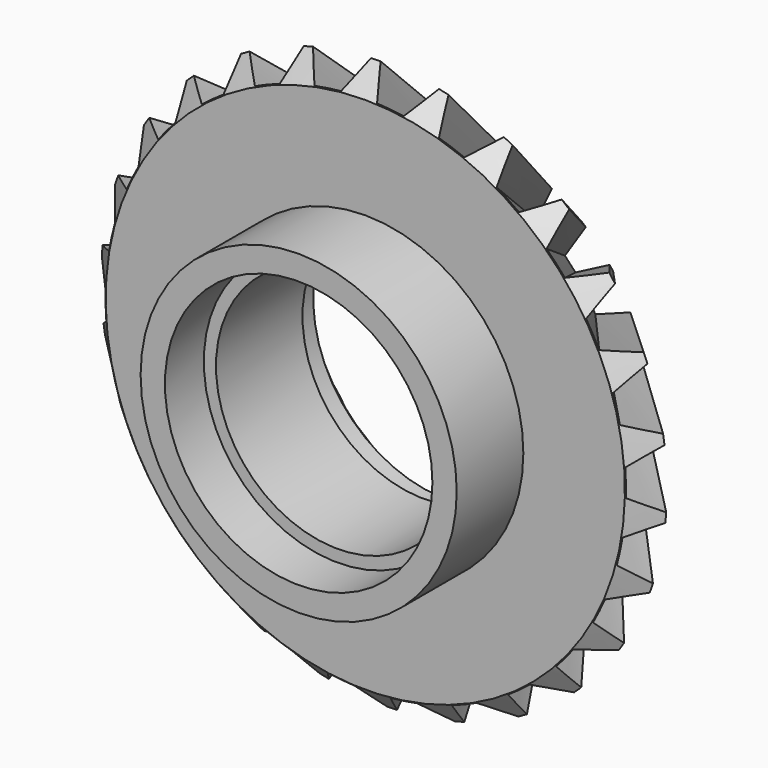
from build123d import *

# Parameters (mm, degrees)
F4_R      = 65
F5_DEPTH  = 34.25
F6_R      = 55
F6_R_2    = 50
F7_DEPTH  = 20
F9_R      = 55
F9_R_2    = 50
F10_DEPTH = 73
F11_DEPTH = 333


# Not quite as in the source:
# - ends of sketch curves that miss each other by under 0.0002 mm in the source are joined


with BuildPart() as f3:
    # F0 (on Front) → F3 section 0
    with BuildSketch(Plane.XZ):
        with BuildLine():
            Line((4.647425, 107.14926), (-1.469582, 125.991429))
            ThreePointArc((-1.469582, 125.991429), (-3.6339068263, 125.9475871987), (-5.7971590014, 125.8665680295))
            Line((-5.7971590014, 125.8665680295), (-10.196493, 106.764198))
            ThreePointArc((-10.196493, 106.764198), (-15.6841394295, 106.0969852086), (-21.1301169921, 105.1478989609))
            Line((-21.1301169921, 105.1478989609), (-31.578602, 121.978653))
            ThreePointArc((-31.578602, 121.978653), (-33.6695433104, 121.4181281904), (-35.7505460521, 120.8217631761))
            Line((-35.7505460521, 120.8217631761), (-35.450546, 101.221644))
            ThreePointArc((-35.450546, 101.221644), (-40.6190569723, 99.2605395446), (-45.6796531382, 97.0357242936))
            Line((-45.6796531382, 97.0357242936), (-59.852387, 110.876921))
            ThreePointArc((-59.852387, 110.876921), (-61.7484272238, 109.8322891293), (-63.626240453, 108.7552367742))
            Line((-63.626240453, 108.7552367742), (-58.644343, 89.796456))
            ThreePointArc((-58.644343, 89.796456), (-63.1933432848, 86.6554318233), (-67.5744545742, 83.2841857077))
            Line((-67.5744545742, 83.2841857077), (-84.64777, 93.331425))
            ThreePointArc((-84.64777, 93.331425), (-86.2387176403, 91.8633963), (-87.8042092574, 90.3682512649))
            Line((-87.8042092574, 90.3682512649), (-78.429944, 73.152624))
            ThreePointArc((-78.429944, 73.152624), (-82.0950620329, 69.0142252714), (-85.5420740481, 64.6924730363))
            Line((-85.5420740481, 64.6924730363), (-104.523732, 70.361846))
            ThreePointArc((-104.523732, 70.361846), (-105.7171271923, 68.5557365814), (-106.8793169138, 66.7293909462))
            Line((-106.8793169138, 66.7293909462), (-93.657481, 52.257427))
            ThreePointArc((-93.657481, 52.257427), (-96.2257139986, 47.3621628039), (-98.5382990262, 42.3410690113))
            Line((-98.5382990262, 42.3410690113), (-118.325154, 43.303093))
            ThreePointArc((-118.325154, 43.303093), (-119.0516411498, 41.2638672394), (-119.7429867773, 39.2124612546))
            Line((-119.7429867773, 39.2124612546), (-103.441986, 28.325219))
            ThreePointArc((-103.441986, 28.325219), (-104.764077079, 22.9575837968), (-105.8078361957, 17.5289560324))
            Line((-105.8078361957, 17.5289560324), (-125.249949, 13.727721))
            ThreePointArc((-125.249949, 13.727721), (-125.4673066239, 11.5738916766), (-125.6476294147, 9.4166460311))
            Line((-125.6476294147, 9.4166460311), (-107.214818, 2.746852))
            ThreePointArc((-107.214818, 2.746852), (-107.2139328185, -2.7812064998), (-106.9282065415, -8.301876042))
            Line((-106.9282065415, -8.301876042), (-124.895671, -16.645457))
            ThreePointArc((-124.895671, -16.645457), (-124.5912682706, -18.7887165799), (-124.2500886239, -20.9264301051))
            Line((-124.2500886239, -20.9264301051), (-104.756715, -22.991152))
            ThreePointArc((-104.756715, -22.991152), (-103.4329044086, -28.3583635916), (-101.8342980115, -33.6502340038))
            Line((-101.8342980115, -33.6502340038), (-117.282912, -46.051261))
            ThreePointArc((-117.282912, -46.051261), (-116.4744381713, -48.0593929703), (-115.6315841333, -50.0533390577))
            Line((-115.6315841333, -50.0533390577), (-96.210533, -47.392994))
            ThreePointArc((-96.210533, -47.392994), (-93.6407315432, -52.2874353555), (-90.8221502197, -57.042962138))
            Line((-90.8221502197, -57.042962138), (-102.854096, -72.780733))
            ThreePointArc((-102.854096, -72.780733), (-101.588537404, -74.537031522), (-100.2929927716, -76.2713288263))
            Line((-100.2929927716, -76.2713288263), (-82.072944, -69.040527))
            ThreePointArc((-82.072944, -69.040527), (-78.4065001697, -73.1777509298), (-74.5317498938, -77.1205598901))
            Line((-74.5317498938, -77.1205598901), (-82.447773, -95.280453))
            ThreePointArc((-82.447773, -95.280453), (-80.7986798888, -96.6828491938), (-79.1257368917, -98.0567068657))
            Line((-79.1257368917, -98.0567068657), (-63.165574, -86.675676))
            ThreePointArc((-63.165574, -86.675676), (-58.6155674419, -89.8152423226), (-53.9098340917, -92.7161921576))
            Line((-53.9098340917, -92.7161921576), (-57.249886, -112.24282))
            ThreePointArc((-57.249886, -112.24282), (-55.3130968687, -113.2098110359), (-53.359980765, -114.1433854972))
            Line((-53.359980765, -114.1433854972), (-40.58725, -99.27355))
            ThreePointArc((-40.58725, -99.27355), (-35.4181109459, -101.2329981628), (-30.1548749802, -102.9234959323))
            Line((-30.1548749802, -102.9234959323), (-28.724843, -122.682042))
            ThreePointArc((-28.724843, -122.682042), (-26.6129171945, -123.1574303012), (-24.4931359084, -123.5964655376))
            Line((-24.4931359084, -123.5964655376), (-15.650143, -106.102006))
            ThreePointArc((-15.650143, -106.102006), (-10.1622832517, -106.7674599263), (-4.6474249612, -107.1492601058))
            Line((-4.6474249612, -107.1492601058), (1.469583, -125.99143))
            ThreePointArc((1.469583, -125.99143), (3.6339078195, -125.9475871701), (5.7971599992, -125.8665679835))
            Line((5.7971599992, -125.8665679835), (10.196493, -106.764199))
            ThreePointArc((10.196493, -106.764199), (15.6841393825, -106.0969852156), (21.1301169921, -105.1478989609))
            Line((21.1301169921, -105.1478989609), (31.578602, -121.978654))
            ThreePointArc((31.578602, -121.978654), (33.6695430529, -121.4181282618), (35.75054578, -120.8217632566))
            Line((35.75054578, -120.8217632566), (35.450547, -101.221645))
            ThreePointArc((35.450547, -101.221645), (40.6190574777, -99.2605393378), (45.6796535714, -97.0357240896))
            Line((45.6796535714, -97.0357240896), (59.852388, -110.876922))
            ThreePointArc((59.852388, -110.876922), (61.7484275564, -109.8322889423), (63.6262407621, -108.7552365934))
            Line((63.6262407621, -108.7552365934), (58.644343, -89.796456))
            ThreePointArc((58.644343, -89.796456), (63.193343344, -86.6554317802), (67.574454688, -83.2841856154))
            Line((67.574454688, -83.2841856154), (84.64777, -93.331426))
            ThreePointArc((84.64777, -93.331426), (86.2387174028, -91.8633965229), (87.804209272, -90.3682512507))
            Line((87.804209272, -90.3682512507), (78.429944, -73.152625))
            ThreePointArc((78.429944, -73.152625), (82.095061541, -69.0142258565), (85.5420735669, -64.6924736725))
            Line((85.5420735669, -64.6924736725), (104.523732, -70.361847))
            ThreePointArc((104.523732, -70.361847), (105.7171267358, -68.5557372853), (106.8793164645, -66.7293916657))
            Line((106.8793164645, -66.7293916657), (93.657481, -52.257428))
            ThreePointArc((93.657481, -52.257428), (96.2257136029, -47.3621636079), (98.5382986635, -42.3410698554))
            Line((98.5382986635, -42.3410698554), (118.325154, -43.303093))
            ThreePointArc((118.325154, -43.303093), (119.0516410451, -41.2638675413), (119.7429865784, -39.212461862))
            Line((119.7429865784, -39.212461862), (103.441986, -28.32522))
            ThreePointArc((103.441986, -28.32522), (104.7640768702, -22.9575847497), (105.8078360344, -17.5289570057))
            Line((105.8078360344, -17.5289570057), (125.249949, -13.727721))
            ThreePointArc((125.249949, -13.727721), (125.4673065815, -11.5738921359), (125.6476293457, -9.416646951))
            Line((125.6476293457, -9.416646951), (107.214819, -2.746853))
            ThreePointArc((107.214819, -2.746853), (107.2139328321, 2.7812059742), (106.9282065475, 8.3018759649))
            Line((106.9282065475, 8.3018759649), (124.895672, 16.645456))
            ThreePointArc((124.895672, 16.645456), (124.5912683668, 18.7887159424), (124.2500886515, 20.9264299413))
            Line((124.2500886515, 20.9264299413), (104.756716, 22.991151))
            ThreePointArc((104.756716, 22.991151), (103.4329046917, 28.3583625593), (101.8342983094, 33.6502331022))
            Line((101.8342983094, 33.6502331022), (117.282912, 46.05126))
            ThreePointArc((117.282912, 46.05126), (116.4744385996, 48.0593919323), (115.6315846557, 50.0533378509))
            Line((115.6315846557, 50.0533378509), (96.210533, 47.392993))
            ThreePointArc((96.210533, 47.392993), (93.6407320979, 52.287434362), (90.822150953, 57.0429609705))
            Line((90.822150953, 57.0429609705), (102.854096, 72.780732))
            ThreePointArc((102.854096, 72.780732), (101.5885378809, 74.537030872), (100.2929932534, 76.2713281927))
            Line((100.2929932534, 76.2713281927), (82.072944, 69.040526))
            ThreePointArc((82.072944, 69.040526), (78.4065004308, 73.17775065), (74.5317498938, 77.1205598901))
            Line((74.5317498938, 77.1205598901), (82.447774, 95.280452))
            ThreePointArc((82.447774, 95.280452), (80.7986806709, 96.6828485402), (79.1257373804, 98.0567064714))
            Line((79.1257373804, 98.0567064714), (63.165574, 86.675675))
            ThreePointArc((63.165574, 86.675675), (58.6155682609, 89.8152417881), (53.9098352735, 92.7161914704))
            Line((53.9098352735, 92.7161914704), (57.249886, 112.242819))
            ThreePointArc((57.249886, 112.242819), (55.3130972631, 113.2098108432), (53.3599811486, 114.1433853179))
            Line((53.3599811486, 114.1433853179), (40.587251, 99.273549))
            ThreePointArc((40.587251, 99.273549), (35.418112147, 101.2329977425), (30.1548761709, 102.9234955834))
            Line((30.1548761709, 102.9234955834), (28.724844, 122.682041))
            ThreePointArc((28.724844, 122.682041), (26.6129183562, 123.1574300502), (24.4931370613, 123.5964653091))
            Line((24.4931370613, 123.5964653091), (15.650144, 106.102005))
            ThreePointArc((15.650144, 106.102005), (10.1622838383, 106.7674598705), (4.647425, 107.14926))
        make_face()
    # F2 (on offset) → F3 section 1
    with BuildSketch(Plane.XZ.offset(-56.5685)):
        with BuildLine():
            Line((-19.7001110751, 66.5780655763), (-18.0915129272, 51.6565431383))
            ThreePointArc((-18.0915129272, 51.6565431383), (-20.7291642653, 50.655730553), (-23.3117433893, 49.5203383384))
            Line((-23.3117433893, 49.5203383384), (-32.9812778687, 61.0980237192))
            ThreePointArc((-32.9812778687, 61.0980237192), (-34.0260786064, 60.5223856678), (-35.0608356411, 59.9288828229))
            Line((-35.0608356411, 59.9288828229), (-29.9280263775, 45.8259154425))
            ThreePointArc((-29.9280263775, 45.8259154425), (-32.2495222328, 44.2229533699), (-34.485339159, 42.502501951))
            Line((-34.485339159, 42.502501951), (-46.6446160079, 51.4296897689))
            ThreePointArc((-46.6446160079, 51.4296897689), (-47.5212975323, 50.6207415305), (-48.3839518806, 49.7968512324))
            Line((-48.3839518806, 49.7968512324), (-40.0252317187, 37.3320521117))
            ThreePointArc((-40.0252317187, 37.3320521117), (-41.8956551903, 35.2200988808), (-43.6547723658, 33.0145746404))
            Line((-43.6547723658, 33.0145746404), (-57.597138611, 38.7724491885))
            ThreePointArc((-57.597138611, 38.7724491885), (-58.2547513786, 37.7772038943), (-58.8951687053, 36.7708076526))
            Line((-58.8951687053, 36.7708076526), (-47.7963160781, 26.6685856085))
            ThreePointArc((-47.7963160781, 26.6685856085), (-49.1069649527, 24.1703802647), (-50.2871488814, 21.6079602549))
            Line((-50.2871488814, 21.6079602549), (-65.2023248751, 23.8618947934))
            ThreePointArc((-65.2023248751, 23.8618947934), (-65.6026508221, 22.7381924823), (-65.9836124001, 21.6077783884))
            Line((-65.9836124001, 21.6077783884), (-52.7896522797, 14.4552378462))
            ThreePointArc((-52.7896522797, 14.4552378462), (-53.4643564085, 11.7159670033), (-53.9970190904, 8.945569761))
            Line((-53.9970190904, 8.945569761), (-69.0181890183, 7.5645738073))
            ThreePointArc((-69.0181890183, 7.5645738073), (-69.1379626558, 6.3777199733), (-69.2373283829, 5.1889835853))
            Line((-69.2373283829, 5.1889835853), (-54.7150457733, 1.4018042029))
            ThreePointArc((-54.7150457733, 1.4018042029), (-54.714593805, -1.4193356746), (-54.568778821, -4.2367047315))
            Line((-54.568778821, -4.2367047315), (-68.8229668866, -9.1723727123))
            ThreePointArc((-68.8229668866, -9.1723727123), (-68.6552274062, -10.3534024386), (-68.4672225075, -11.5313760825))
            Line((-68.4672225075, -11.5313760825), (-53.4605996877, -11.7330972054))
            ThreePointArc((-53.4605996877, -11.7330972054), (-52.7850178889, -14.4721517221), (-51.969199476, -17.1727573448))
            Line((-51.969199476, -17.1727573448), (-64.6280040808, -25.3762542701))
            ThreePointArc((-64.6280040808, -25.3762542701), (-64.1824998913, -26.4828227338), (-63.7180505282, -27.5815740873))
            Line((-63.7180505282, -27.5815740873), (-49.0992178696, -24.1861136521))
            ThreePointArc((-49.0992178696, -24.1861136521), (-47.7877685989, -26.6838989156), (-46.3493591578, -29.1107917217))
            Line((-46.3493591578, -29.1107917217), (-56.6770965911, -40.1053601686))
            ThreePointArc((-56.6770965911, -40.1053601686), (-55.9797187767, -41.0731576329), (-55.2658170579, -42.0288312611))
            Line((-55.2658170579, -42.0288312611), (-41.8843679773, -35.2335210863))
            ThreePointArc((-41.8843679773, -35.2335210863), (-40.0132678994, -37.3448748962), (-38.0358625584, -39.3570126971))
            Line((-38.0358625584, -39.3570126971), (-45.4323222603, -52.5036883112))
            ThreePointArc((-45.4323222603, -52.5036883112), (-44.5235998847, -53.2764699051), (-43.6017351833, -54.0335255305))
            Line((-43.6017351833, -54.0335255305), (-32.2353508617, -44.2332843436))
            ThreePointArc((-32.2353508617, -44.2332843436), (-29.9133415119, -45.8355024909), (-27.5118598818, -47.3159471515))
            Line((-27.5118598818, -47.3159471515), (-31.5471864996, -61.8506929323))
            ThreePointArc((-31.5471864996, -61.8506929323), (-30.4799312042, -62.3835473986), (-29.4036789456, -62.8979877))
            Line((-29.4036789456, -62.8979877), (-20.7129323247, -50.6623698963))
            ThreePointArc((-20.7129323247, -50.6623698963), (-18.0749604462, -51.6623372861), (-15.3889679105, -52.5250507439))
            Line((-15.3889679105, -52.5250507439), (-15.8286429288, -67.6031600983))
            ThreePointArc((-15.8286429288, -67.6031600983), (-14.6648797121, -67.8651198723), (-13.4967877657, -68.1070474493))
            Line((-13.4967877657, -68.1070474493), (-7.9867534495, -54.1471426609))
            ThreePointArc((-7.9867534495, -54.1471426609), (-5.1861283793, -54.4867448232), (-2.3717250608, -54.6815893079))
            Line((-2.3717250608, -54.6815893079), (0.8098038342, -69.4267773269))
            ThreePointArc((0.8098038342, -69.4267773269), (2.0024412842, -69.4026182586), (3.1944876603, -69.3579731598))
            Line((3.1944876603, -69.3579731598), (5.2035865056, -54.4850803108))
            ThreePointArc((5.2035865056, -54.4850803108), (8.0041026182, -54.1445808025), (10.7833538285, -53.6602326608))
            Line((10.7833538285, -53.6602326608), (17.4011877418, -67.2155626133))
            ThreePointArc((17.4011877418, -67.2155626133), (18.5533876716, -66.90668874), (19.7001110751, -66.5780655763))
            Line((19.7001110751, -66.5780655763), (18.0915129272, -51.6565431383))
            ThreePointArc((18.0915129272, -51.6565431383), (20.7291642653, -50.655730553), (23.3117433893, -49.5203383384))
            Line((23.3117433893, -49.5203383384), (32.9812778687, -61.0980237192))
            ThreePointArc((32.9812778687, -61.0980237192), (34.0260786064, -60.5223856678), (35.0608356411, -59.9288828229))
            Line((35.0608356411, -59.9288828229), (29.9280263775, -45.8259154425))
            ThreePointArc((29.9280263775, -45.8259154425), (32.2495222328, -44.2229533699), (34.485339159, -42.502501951))
            Line((34.485339159, -42.502501951), (46.6446160079, -51.4296897689))
            ThreePointArc((46.6446160079, -51.4296897689), (47.5212975323, -50.6207415305), (48.3839518806, -49.7968512324))
            Line((48.3839518806, -49.7968512324), (40.0252317187, -37.3320521117))
            ThreePointArc((40.0252317187, -37.3320521117), (41.8956551903, -35.2200988808), (43.6547723658, -33.0145746404))
            Line((43.6547723658, -33.0145746404), (57.597138611, -38.7724491885))
            ThreePointArc((57.597138611, -38.7724491885), (58.2547513786, -37.7772038943), (58.8951687053, -36.7708076526))
            Line((58.8951687053, -36.7708076526), (47.7963160781, -26.6685856085))
            ThreePointArc((47.7963160781, -26.6685856085), (49.1069649527, -24.1703802647), (50.2871488814, -21.6079602549))
            Line((50.2871488814, -21.6079602549), (65.2023248751, -23.8618947934))
            ThreePointArc((65.2023248751, -23.8618947934), (65.6026508221, -22.7381924823), (65.9836124001, -21.6077783884))
            Line((65.9836124001, -21.6077783884), (52.7896522797, -14.4552378462))
            ThreePointArc((52.7896522797, -14.4552378462), (53.4643564085, -11.7159670033), (53.9970190904, -8.945569761))
            Line((53.9970190904, -8.945569761), (69.0181890183, -7.5645738073))
            ThreePointArc((69.0181890183, -7.5645738073), (69.1379626558, -6.3777199733), (69.2373283829, -5.1889835853))
            Line((69.2373283829, -5.1889835853), (54.7150457733, -1.4018042029))
            ThreePointArc((54.7150457733, -1.4018042029), (54.714593805, 1.4193356746), (54.568778821, 4.2367047315))
            Line((54.568778821, 4.2367047315), (68.8229668866, 9.1723727123))
            ThreePointArc((68.8229668866, 9.1723727123), (68.6552274062, 10.3534024386), (68.4672225075, 11.5313760825))
            Line((68.4672225075, 11.5313760825), (53.4605996877, 11.7330972054))
            ThreePointArc((53.4605996877, 11.7330972054), (52.7850178889, 14.4721517221), (51.969199476, 17.1727573448))
            Line((51.969199476, 17.1727573448), (64.6280040808, 25.3762542701))
            ThreePointArc((64.6280040808, 25.3762542701), (64.1824998913, 26.4828227338), (63.7180505282, 27.5815740873))
            Line((63.7180505282, 27.5815740873), (49.0992178696, 24.1861136521))
            ThreePointArc((49.0992178696, 24.1861136521), (47.7877685989, 26.6838989156), (46.3493591578, 29.1107917217))
            Line((46.3493591578, 29.1107917217), (56.6770965911, 40.1053601686))
            ThreePointArc((56.6770965911, 40.1053601686), (55.9797187767, 41.0731576329), (55.2658170579, 42.0288312611))
            Line((55.2658170579, 42.0288312611), (41.8843679773, 35.2335210863))
            ThreePointArc((41.8843679773, 35.2335210863), (40.0132678994, 37.3448748962), (38.0358625584, 39.3570126971))
            Line((38.0358625584, 39.3570126971), (45.4323222603, 52.5036883112))
            ThreePointArc((45.4323222603, 52.5036883112), (44.5235998847, 53.2764699051), (43.6017351833, 54.0335255305))
            Line((43.6017351833, 54.0335255305), (32.2353508617, 44.2332843436))
            ThreePointArc((32.2353508617, 44.2332843436), (29.9133415119, 45.8355024909), (27.5118598818, 47.3159471515))
            Line((27.5118598818, 47.3159471515), (31.5471864996, 61.8506929323))
            ThreePointArc((31.5471864996, 61.8506929323), (30.4799312042, 62.3835473986), (29.4036789456, 62.8979877))
            Line((29.4036789456, 62.8979877), (20.7129323247, 50.6623698963))
            ThreePointArc((20.7129323247, 50.6623698963), (18.0749604462, 51.6623372861), (15.3889679105, 52.5250507439))
            Line((15.3889679105, 52.5250507439), (15.8286429288, 67.6031600983))
            ThreePointArc((15.8286429288, 67.6031600983), (14.6648797121, 67.8651198723), (13.4967877657, 68.1070474493))
            Line((13.4967877657, 68.1070474493), (7.9867534495, 54.1471426609))
            ThreePointArc((7.9867534495, 54.1471426609), (5.1861283793, 54.4867448232), (2.3717250608, 54.6815893079))
            Line((2.3717250608, 54.6815893079), (-0.8098038342, 69.4267773269))
            ThreePointArc((-0.8098038342, 69.4267773269), (-2.0024412842, 69.4026182586), (-3.1944876603, 69.3579731598))
            Line((-3.1944876603, 69.3579731598), (-5.2035865056, 54.4850803108))
            ThreePointArc((-5.2035865056, 54.4850803108), (-8.0041026182, 54.1445808025), (-10.7833538285, 53.6602326608))
            Line((-10.7833538285, 53.6602326608), (-17.4011877418, 67.2155626133))
            ThreePointArc((-17.4011877418, 67.2155626133), (-18.5533876716, 66.90668874), (-19.7001110751, 66.5780655763))
        make_face()
    loft()

    # F4 (on face) → F5 (join)
    with BuildSketch(Plane.XZ):
        Circle(F4_R)
    extrude(amount=F5_DEPTH)

    # F6 (on face) → F7 (cut)
    with BuildSketch(Plane.XZ.offset(34.25)):
        Circle(F6_R)
        Circle(F6_R_2, mode=Mode.SUBTRACT)
    extrude(amount=-F7_DEPTH, mode=Mode.SUBTRACT)

    # F9 (on offset) → F10 (cut)
    with BuildSketch(Plane.XZ.offset(-30.213)):
        Circle(F9_R)
        Circle(F9_R_2, mode=Mode.SUBTRACT)
    extrude(amount=-F10_DEPTH, mode=Mode.SUBTRACT)

    # F11 (cut): a face of the model
    f11_faces = [f3.faces().sort_by_distance(p)[0] for p in [
        (0, -34.25, 0),
    ]]
    extrude(f11_faces, amount=-F11_DEPTH, mode=Mode.SUBTRACT)

    # F12 (on Right) → F13 (revolve, cut)
    with BuildSketch(Plane.YZ):
        Polygon((56.6436164081, 54.7567647678), (56.6436164081, 69.6557834744), (41.7445977015, 54.7567647678), align=None)
        Polygon((0, 129.4315974777), (0, 106.764198), (22.6673994777, 129.4315974777), align=None)
    revolve(axis=Axis((0, -34.25, 0), (0, -1, 0)), mode=Mode.SUBTRACT)


solid = f3.part
